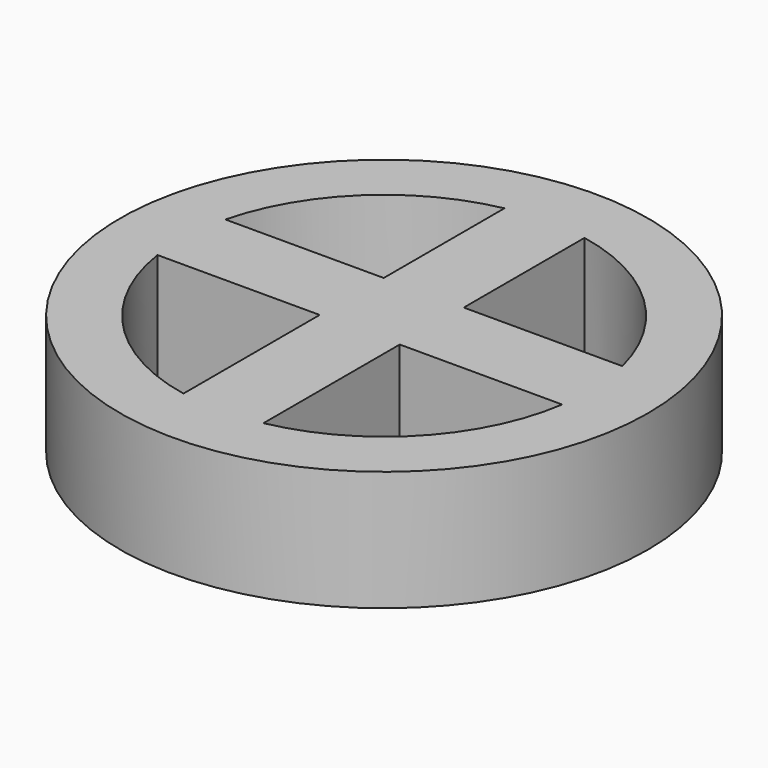
from build123d import *

# Parameters (mm, degrees)
F0_R     = 83.7442407906
F1_DEPTH = 38.1
F3_DEPTH = 50.8


with BuildPart() as f1:
    # F0 (on Top) → F1 (new body)
    with BuildSketch(Plane.XY):
        Circle(F0_R)
    extrude(amount=F1_DEPTH)

    # F2 (on face) → F3 (cut)
    with BuildSketch(Plane.XY.offset(38.1)):
        with BuildLine():
            Line((12.6646681265, 15.7748187695), (62.9699063944, 15.7748187695))
            ThreePointArc((62.9699063944, 15.7748187695), (44.7615355408, 47.0155182314), (12.6646681265, 63.6683610578))
            Line((12.6646681265, 63.6683610578), (12.6646681265, 15.7748187695))
        make_face()
        with BuildLine():
            ThreePointArc((12.6646681265, -63.6683610578), (46.9802272386, -44.7985743874), (64.1982079564, -9.6251812305))
            Line((64.1982079564, -9.6251812305), (12.6646681265, -9.6251812305))
            Line((12.6646681265, -9.6251812305), (12.6646681265, -63.6683610578))
        make_face()
        with BuildLine():
            Line((-12.7353318735, 15.7748187695), (-12.7353318735, 63.6542641196))
            ThreePointArc((-12.7353318735, 63.6542641196), (-44.7876221412, 46.990668451), (-62.9699063944, 15.7748187695))
            Line((-62.9699063944, 15.7748187695), (-12.7353318735, 15.7748187695))
        make_face()
        with BuildLine():
            ThreePointArc((-64.1982079564, -9.6251812305), (-47.0050830991, -44.7724935801), (-12.7353318735, -63.6542641196))
            Line((-12.7353318735, -63.6542641196), (-12.7353318735, -9.6251812305))
            Line((-12.7353318735, -9.6251812305), (-64.1982079564, -9.6251812305))
        make_face()
    extrude(amount=-F3_DEPTH, mode=Mode.SUBTRACT)


solid = f1.part
